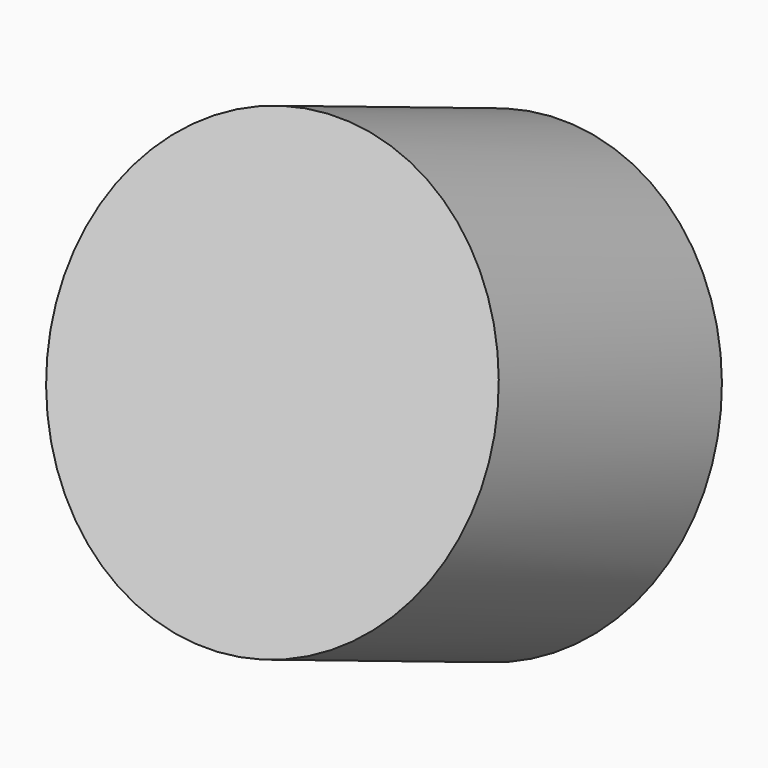
from build123d import *

# Parameters (mm, degrees)
F4_DEPTH     = 31.75
F6_DEPTH     = 80.772
F7_W         = 115.0478571653
F7_H         = 280.0295129418
F8_DEPTH     = 80.01
F10_R        = 5.08
F11_R        = 5.08
F12_R        = 1.27
F13_T4_DEPTH = 185.7457951761
F13_T9_DEPTH = 185.7457951761
F15_R        = 18.2048484519
F16_DEPTH    = 25.4


# Not quite as in the source:
# - a fillet or chamfer that OpenCascade refuses, or shapes differently, is made with other operations: its cross-section is extruded or revolved along the edge and cut away or added
# - a feature of the source that left no trace in its solid (it failed there, or was rolled back) is left out


with BuildPart() as f4:
    # F3 (on Right) → F4 (new body, symmetric)
    with BuildSketch(Plane.YZ):
        Polygon((33.4092862904, 0), (34.8578840494, 0), (34.8578840494, 165.3004437685), (51.5383556485, 200.2867460251), (45.9728437156, 202.9402234647), (21.1225822568, 165.3004437685), align=None)
    extrude(amount=F4_DEPTH, both=True)

    # F5 (on Front) → F6 (cut, symmetric)
    with BuildSketch(Plane.XZ):
        Polygon((-36.7620885372, 0), (-2.4731955491, 0), (-9.2842681333, 165.0800704956), (-36.7620885372, 165.0800704956), align=None)
    extrude(amount=F6_DEPTH, both=True, mode=Mode.SUBTRACT)

    # F7 (on Front) → F8 (cut)
    with BuildSketch(Plane.XZ):
        with Locations((57.5239285827, 90.4524587095)):
            Rectangle(F7_W, F7_H)
    extrude(amount=-F8_DEPTH, mode=Mode.SUBTRACT)

    # F9: F4 across face


with BuildPart() as f4_1:
    add(f4.part)
    add(f4.part.mirror(Plane(origin=(0, 31.8435446529, 122.6723093361), x_dir=(0, 1, 0), z_dir=(1, 0, 0))))

    # F10
    f10_edges = [f4_1.edges().sort_by_distance(p)[0] for p in [
        (-9.284268, 27.998423, 165.08007),
        (9.284268, 27.998423, 165.08007),
        (31.75, 27.998423, 165.08007),
        (-31.75, 27.998423, 165.08007),
    ]]
    fillet(f10_edges, radius=F10_R)

    # F11
    f11_edges = [f4_1.edges().sort_by_distance(p)[0] for p in [
        (-31.75, 48.7556, 201.613485),
        (31.75, 48.7556, 201.613485),
    ]]
    fillet(f11_edges, radius=F11_R)

    # F12
    f12_edges = [f4_1.edges().sort_by_distance(p)[0] for p in [
        (-31.75, 33.738898, 184.409914),
    ]]
    fillet(f12_edges, radius=F12_R)

    # F13: fillet of radius 5.08 on 2 edges, made by hand


with BuildPart() as f13_tool2:
    # F13_s3 → F13_t4 (new body)
    with BuildSketch(Plane(origin=(7.1378657639, 0, 173.0005617946), x_dir=(0, 1, 0), z_dir=(-0.0412241322, 0, -0.9991499241))):
        with BuildLine():
            ThreePointArc((29.7778840494, 2.4710931453), (33.3699864978, 0.9831955937), (34.8578840494, -2.6089068547))
            Line((34.8578840494, -2.6089068547), (34.8578840494, 2.4710931453))
            Line((34.8578840494, 2.4710931453), (29.7778840494, 2.4710931453))
        make_face()
    extrude(amount=F13_T4_DEPTH)

    split(bisect_by=Plane(origin=(0, -35.8121563615, 17.0742152946), x_dir=(1, 0, 0), z_dir=(0, 0.902656838, -0.4303610493)), keep=Keep.TOP)


with BuildPart() as f4_2:
    add(f4_1.part)

    # F13_t1: cut F13_tool2
    add(f13_tool2.part, mode=Mode.SUBTRACT)


with BuildPart() as f13_tool7:
    # F13_s8 → F13_t9 (new body)
    with BuildSketch(Plane(origin=(-7.1378657639, 0, 173.0005617946), x_dir=(0, 1, 0), z_dir=(0.0412241322, 0, -0.9991499241))):
        with BuildLine():
            ThreePointArc((29.7778840494, -2.4710931453), (33.3699864978, -0.9831955937), (34.8578840494, 2.6089068547))
            Line((34.8578840494, 2.6089068547), (34.8578840494, -2.4710931453))
            Line((34.8578840494, -2.4710931453), (29.7778840494, -2.4710931453))
        make_face()
    extrude(amount=F13_T9_DEPTH)

    split(bisect_by=Plane(origin=(0, -35.8121563615, 17.0742152946), x_dir=(1, 0, 0), z_dir=(0, 0.902656838, -0.4303610493)), keep=Keep.TOP)


with BuildPart() as f4_3:
    add(f4_2.part)

    # F13_t6: cut F13_tool7
    add(f13_tool7.part, mode=Mode.SUBTRACT)


with BuildPart() as f16:
    # F15 (on line) → F16 (new body)
    with BuildSketch(Plane(origin=(0, -63.794974886, 26.4515642177), x_dir=(-1, 0, 0), z_dir=(0, 0.9237421686, -0.3830148901))):
        with Locations((-38.6807657778, 154.1410535574)):
            Circle(F15_R)
    extrude(amount=F16_DEPTH)


solid = f16.part
